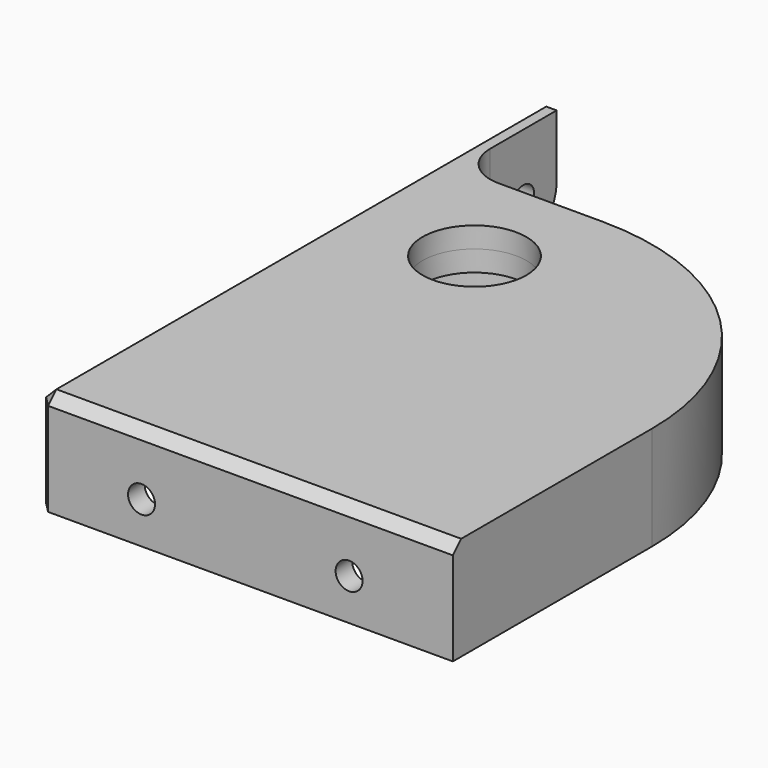
from build123d import *

# Parameters (mm, degrees)
F0_R      = 21
F0_R_2    = 12.5
F1_DEPTH  = 5
F2_DEPTH  = 20
F3_W      = 5
F3_H      = 25
F4_DEPTH  = 30
F6_R      = 3.25
F7_DEPTH  = 25
F5_R      = 3
F5_R_2    = 3.25
F8_DEPTH  = 25
F9_SIZE   = 2.5
F10_R     = 10
F11_DEPTH = 5
F12_SIZE  = 1


# Not quite as in the source:
# - a feature names something its author has since deleted; it is built from what else it names


with BuildPart() as f1:
    # F0 (on Top) → F1 (new body)
    with BuildSketch(Plane.XY):
        with BuildLine():
            Line((30, 65), (5, 65))
            Line((5, 65), (5, 5))
            Line((5, 5), (95, 5))
            Line((95, 5), (95, 61.8416720113))
            ThreePointArc((95, 61.8416720113), (89.0121465356, 85.9307991151), (72.4423646792, 104.4127568838))
            ThreePointArc((72.4423646792, 104.4127568838), (64.4445964825, 104.6534027902), (60, 98))
            Line((60, 98), (60, 95))
            ThreePointArc((60, 95), (51.2132034356, 73.7867965644), (30, 65))
        make_face()
        with BuildLine():
            Line((40, 120), (5, 120))
            Line((5, 120), (5, 65))
            Line((5, 65), (30, 65))
            ThreePointArc((30, 65), (51.2132034356, 73.7867965644), (60, 95))
            Line((60, 95), (60, 98))
            ThreePointArc((60, 98), (64.4445964825, 104.6534027902), (72.4423646792, 104.4127568838))
            ThreePointArc((72.4423646792, 104.4127568838), (89.0121465356, 85.9307991151), (95, 61.8416720113))
            Line((95, 61.8416720113), (95, 5))
            Line((95, 5), (100, 5))
            Line((100, 5), (100, 60))
            ThreePointArc((100, 60), (82.4264068712, 102.4264068712), (40, 120))
        make_face()
        with Locations((30, 94)):
            Circle(F0_R, mode=Mode.SUBTRACT)
        with Locations((30, 94)):
            Circle(F0_R)
        with Locations((30, 94)):
            Circle(F0_R_2, mode=Mode.SUBTRACT)
        Polygon((0, 120), (0, 0), (100, 0), (100, 5), (95, 5), (5, 5), (5, 65), (5, 120), align=None)
    extrude(amount=F1_DEPTH)

    # F0 (on Top) → F2 (join)
    with BuildSketch(Plane.XY):
        Polygon((0, 120), (0, 0), (100, 0), (100, 5), (95, 5), (5, 5), (5, 65), (5, 120), align=None)
        with BuildLine():
            Line((40, 120), (5, 120))
            Line((5, 120), (5, 65))
            Line((5, 65), (30, 65))
            ThreePointArc((30, 65), (51.2132034356, 73.7867965644), (60, 95))
            Line((60, 95), (60, 98))
            ThreePointArc((60, 98), (64.4445964825, 104.6534027902), (72.4423646792, 104.4127568838))
            ThreePointArc((72.4423646792, 104.4127568838), (89.0121465356, 85.9307991151), (95, 61.8416720113))
            Line((95, 61.8416720113), (95, 5))
            Line((95, 5), (100, 5))
            Line((100, 5), (100, 60))
            ThreePointArc((100, 60), (82.4264068712, 102.4264068712), (40, 120))
        make_face()
        with Locations((30, 94)):
            Circle(F0_R, mode=Mode.SUBTRACT)
    extrude(amount=-F2_DEPTH)

    # F3 (on face) → F4 (join)
    with BuildSketch(Plane(origin=(0, 120, 0), x_dir=(-1, 0, 0), z_dir=(0, 1, 0))):
        with Locations((-2.5, -7.5)):
            Rectangle(F3_W, F3_H)
    extrude(amount=F4_DEPTH)

    # F6 (on face) → F7 (cut)
    with BuildSketch(Plane.XZ):
        with Locations((25, -10)):
            Circle(F6_R)
        with Locations((75, -10)):
            Circle(F6_R)
    extrude(amount=-F7_DEPTH, mode=Mode.SUBTRACT)

    # F5 (on face) → F8 (cut)
    with BuildSketch(Plane(origin=(0, 0, 0), x_dir=(0, -1, 0), z_dir=(-1, 0, 0))):
        with Locations((-25, -10)):
            Circle(F5_R)
        with Locations((-140, -10)):
            Circle(F5_R_2)
    extrude(amount=-F8_DEPTH, mode=Mode.SUBTRACT)

    # F9
    f9_edges = [f1.edges().sort_by_distance(p)[0] for p in [
        (50, 0, 5),
        (0, 75, 5),
        (0, 0, -7.5),
    ]]
    chamfer(f9_edges, length=F9_SIZE)

    # F10
    f10_edges = [f1.edges().sort_by_distance(p)[0] for p in [
        (5, 5, -10),
        (95, 5, -10),
        (5, 65, -10),
        (5, 120, -7.5),
        (2.5, 150, -20),
    ]]
    fillet(f10_edges, radius=F10_R)

    # F0 (on Top) → F11 (join)
    with BuildSketch(Plane.XY):
        with Locations((30, 94)):
            Circle(F0_R)
        with Locations((30, 94)):
            Circle(F0_R_2, mode=Mode.SUBTRACT)
    extrude(amount=-F11_DEPTH)

    # F12
    f12_edges = [f1.edges().sort_by_distance(p)[0] for p in [
        (9, 94, -20),
    ]]
    chamfer(f12_edges, length=F12_SIZE)


solid = f1.part
